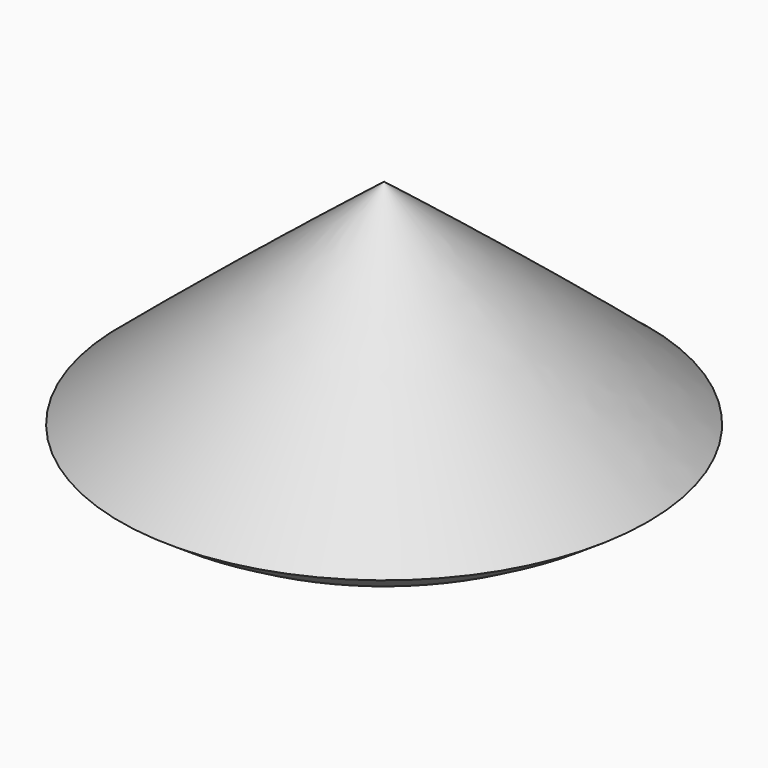
from build123d import *


with BuildPart() as f1:
    # F0 (on Front) → F1 (revolve)
    with BuildSketch(Plane.XZ):
        with BuildLine():
            add(Edge.make_bspline(
                [(-13.569127879, 44.1086594113), (-15.2229193766, 45.4923734906), (-16.8594223359, 46.8165619182), (-18.4664335102, 48.0712763965)],
                knots=[0.9790027247, 0.9790027247, 0.9790027247, 0.9790027247, 1, 1, 1, 1], degree=3))
            Line((-18.4664335102, 48.0712763965), (-18.4664335102, 42.5271638013))
            ThreePointArc((-18.4664335102, 42.5271638013), (-15.8932676192, 42.9323407699), (-13.569127879, 44.1086594113))
        make_face()
    revolve(axis=Axis((-18.4664335102, 0, -6.7288363023), (0, 0, -1)))


solid = f1.part
